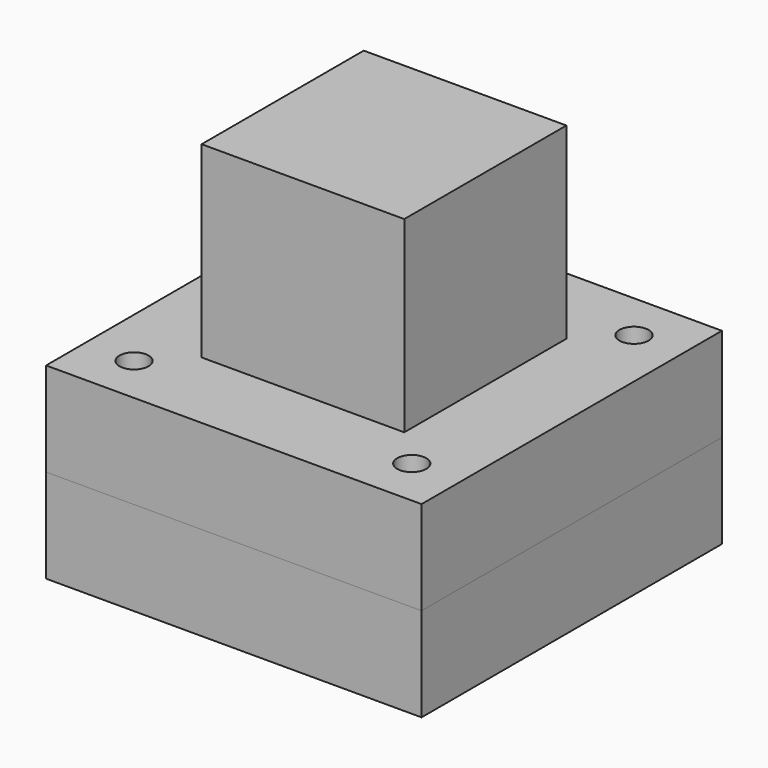
from build123d import *

# Parameters (mm, degrees)
F0_W     = 80
F0_H     = 80
F1_DEPTH = 10
F0_R     = 3
F2_W     = 80
F2_H     = 80
F2_R     = 3
F3_DEPTH = 20
F4_W     = 80
F4_H     = 80
F5_DEPTH = 10
F6_W     = 43.18
F6_H     = 43.18
F6_R     = 1.5
F6_R_2   = 3
F7_DEPTH = 40
F6_R_3   = 3.1
F8_DEPTH = 25


with BuildPart() as f1:
    # F0 (on Top) → F1 (new body)
    with BuildSketch(Plane.XY):
        Rectangle(F0_W, F0_H)
        with BuildLine():
            ThreePointArc((-24.7487373417, -24.7487373413), (-35, 1.228e-07), (-24.7487371681, 24.748737515))
            ThreePointArc((-24.7487371681, 24.748737515), (1.227e-07, 35), (24.7487373415, 24.7487373415))
            ThreePointArc((24.7487373415, 24.7487373415), (32.3357836379, 13.3939201328), (35, 0))
            ThreePointArc((35, 0), (32.3357836202, -13.3939201755), (24.7487372761, -24.7487374069))
            ThreePointArc((24.7487372761, -24.7487374069), (-4.64e-08, -35), (-24.7487373417, -24.7487373413))
        make_face(mode=Mode.SUBTRACT)
    extrude(amount=-F1_DEPTH)

    # F4 (on face) → F5 (join)
    with BuildSketch(Plane.XY):
        Rectangle(F4_W, F4_H)
    extrude(amount=F5_DEPTH)

    # F6 (on face) → F8 (cut)
    with BuildSketch(Plane.XY.offset(10)):
        with Locations((19.59, -19.59)):
            Circle(F6_R)
        with Locations((-19.59, -19.59)):
            Circle(F6_R)
        with Locations((-19.59, 19.59)):
            Circle(F6_R)
        with Locations((19.59, 19.59)):
            Circle(F6_R)
        Circle(F6_R_2)
        with Locations((-29.59, -29.59)):
            Circle(F6_R_3)
        with Locations((29.59, -29.59)):
            Circle(F6_R_3)
        with Locations((-29.59, 29.59)):
            Circle(F6_R_3)
        with Locations((29.59, 29.59)):
            Circle(F6_R_3)
    extrude(amount=-F8_DEPTH, mode=Mode.SUBTRACT)


with BuildPart() as f1b:
    # F0 (on Top) → F1, piece 2 (new body)
    with BuildSketch(Plane.XY):
        with BuildLine():
            ThreePointArc((-8.2495791516, 8.2495790761), (-5.7205636919, 12.0345181588), (-4.832491561, 16.4991582277))
            ThreePointArc((-4.832491561, 16.4991582277), (-12.0345180701, 27.2777527267), (-24.7487371681, 24.748737515))
            ThreePointArc((-24.7487371681, 24.748737515), (-24.7487374471, 8.2495792195), (-8.2495791516, 8.2495790761))
        make_face()
        with Locations((-16.4991582277, 16.4991582277)):
            Circle(F0_R, mode=Mode.SUBTRACT)
    extrude(amount=-F1_DEPTH)


with BuildPart() as f1c:
    # F0 (on Top) → F1, piece 3 (new body)
    with BuildSketch(Plane.XY):
        with BuildLine():
            ThreePointArc((28.1658248944, 16.4991582277), (27.2777527737, 20.9637982719), (24.7487373415, 24.7487373415))
            ThreePointArc((24.7487373415, 24.7487373415), (8.24957912, 24.7487373477), (8.2495791015, 8.2495791262))
            ThreePointArc((8.2495791015, 8.2495791262), (20.9637982639, 5.7205636784), (28.1658248944, 16.4991582277))
        make_face()
        with Locations((16.4991582277, 16.4991582277)):
            Circle(F0_R, mode=Mode.SUBTRACT)
    extrude(amount=-F1_DEPTH)


with BuildPart() as f1d:
    # F0 (on Top) → F1, piece 4 (new body)
    with BuildSketch(Plane.XY):
        with BuildLine():
            ThreePointArc((-8.2495791138, -8.2495791138), (-24.7487373414, -8.2495791137), (-24.7487373417, -24.7487373413))
            ThreePointArc((-24.7487373417, -24.7487373413), (-12.0345181836, -27.2777527737), (-4.832491561, -16.4991582277))
            ThreePointArc((-4.832491561, -16.4991582277), (-5.7205636817, -12.0345181834), (-8.2495791138, -8.2495791138))
        make_face()
        with Locations((-16.4991582277, -16.4991582277)):
            Circle(F0_R, mode=Mode.SUBTRACT)
    extrude(amount=-F1_DEPTH)


with BuildPart() as f1e:
    # F0 (on Top) → F1, piece 5 (new body)
    with BuildSketch(Plane.XY):
        with BuildLine():
            ThreePointArc((8.2495791392, -8.2495790884), (8.2495790684, -24.7487372961), (24.7487372761, -24.7487374069))
            ThreePointArc((24.7487372761, -24.7487374069), (27.277752756, -20.9637983147), (28.1658248944, -16.4991582277))
            ThreePointArc((28.1658248944, -16.4991582277), (20.9637982885, -5.7205636886), (8.2495791392, -8.2495790884))
        make_face()
        with Locations((16.4991582277, -16.4991582277)):
            Circle(F0_R, mode=Mode.SUBTRACT)
    extrude(amount=-F1_DEPTH)


with BuildPart() as f1f:
    # F0 (on Top) → F1, piece 6 (new body)
    with BuildSketch(Plane.XY):
        with BuildLine():
            ThreePointArc((8.2495791015, 8.2495791262), (-3.54e-08, 11.6666666667), (-8.2495791516, 8.2495790761))
            ThreePointArc((-8.2495791516, 8.2495790761), (-11.6666666667, -2.67e-08), (-8.2495791138, -8.2495791138))
            ThreePointArc((-8.2495791138, -8.2495791138), (1.8e-08, -11.6666666667), (8.2495791392, -8.2495790884))
            ThreePointArc((8.2495791392, -8.2495790884), (10.7785945528, -4.4646400277), (11.6666666667, 0))
            ThreePointArc((11.6666666667, 0), (10.7785945426, 4.4646400523), (8.2495791015, 8.2495791262))
        make_face()
        Circle(F0_R, mode=Mode.SUBTRACT)
    extrude(amount=-F1_DEPTH)


with BuildPart() as f3:
    # F2 (on face) → F3 (new body)
    with BuildSketch(Plane(origin=(0, 0, -10), x_dir=(1, 0, 0), z_dir=(0, 0, -1))):
        Rectangle(F2_W, F2_H)
        with Locations((-16.4991582277, -16.4991582277)):
            Circle(F2_R, mode=Mode.SUBTRACT)
        with Locations((16.4991582277, -16.4991582277)):
            Circle(F2_R, mode=Mode.SUBTRACT)
        with Locations((-16.4991582277, 16.4991582277)):
            Circle(F2_R, mode=Mode.SUBTRACT)
        with Locations((16.4991582277, 16.4991582277)):
            Circle(F2_R, mode=Mode.SUBTRACT)
    extrude(amount=F3_DEPTH)


with BuildPart() as f7:
    # F6 (on face) → F7 (new body)
    with BuildSketch(Plane.XY.offset(10)):
        Rectangle(F6_W, F6_H)
        with Locations((-19.59, -19.59)):
            Circle(F6_R, mode=Mode.SUBTRACT)
        with Locations((19.59, -19.59)):
            Circle(F6_R, mode=Mode.SUBTRACT)
        with Locations((-19.59, 19.59)):
            Circle(F6_R, mode=Mode.SUBTRACT)
        Circle(F6_R_2, mode=Mode.SUBTRACT)
        with Locations((19.59, 19.59)):
            Circle(F6_R, mode=Mode.SUBTRACT)
        Circle(F6_R_2)
        with Locations((19.59, -19.59)):
            Circle(F6_R)
        with Locations((-19.59, -19.59)):
            Circle(F6_R)
        with Locations((-19.59, 19.59)):
            Circle(F6_R)
        with Locations((19.59, 19.59)):
            Circle(F6_R)
    extrude(amount=F7_DEPTH)


solid = Compound([f1.part, f1b.part, f1c.part, f1d.part, f1e.part, f1f.part, f3.part, f7.part])
